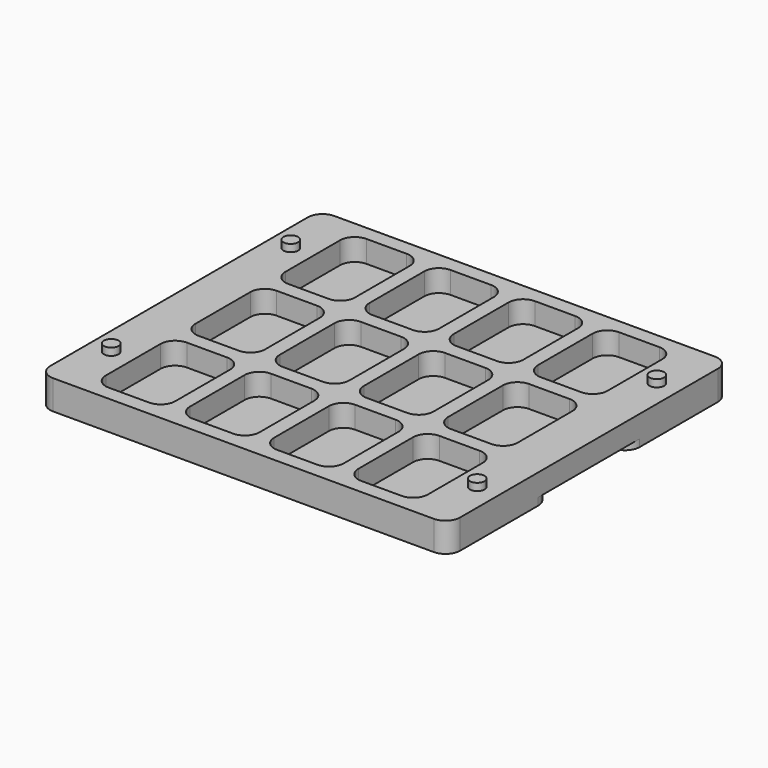
from build123d import *

# Parameters (mm, degrees)
F0_R     = 6.35
F1_DEPTH = 19.05
F2_DEPTH = 6.35
F3_DEPTH = 25.4


# Not quite as in the source:
# - a feature names something its author has since deleted; it is built from what else it names


with BuildPart() as f1:
    # F0 (on Top) → F1 (new body)
    with BuildSketch(Plane.XY):
        with BuildLine():
            Line((-165.1, -152.4), (165.1, -152.4))
            ThreePointArc((165.1, -152.4), (174.0802561211, -148.6802561211), (177.8, -139.7))
            Line((177.8, -139.7), (177.8, -55.0333333333))
            ThreePointArc((177.8, -55.0333333333), (174.0802561211, -46.0530772123), (165.1, -42.3333333333))
            ThreePointArc((165.1, -42.3333333333), (156.1197438789, -38.6135894544), (152.4, -29.6333333333))
            Line((152.4, -29.6333333333), (152.4, 29.6333333333))
            ThreePointArc((152.4, 29.6333333333), (156.1197438789, 38.6135894544), (165.1, 42.3333333333))
            ThreePointArc((165.1, 42.3333333333), (174.0802561211, 46.0530772123), (177.8, 55.0333333333))
            Line((177.8, 55.0333333333), (177.8, 139.7))
            ThreePointArc((177.8, 139.7), (174.0802561211, 148.6802561211), (165.1, 152.4))
            Line((165.1, 152.4), (-165.1, 152.4))
            ThreePointArc((-165.1, 152.4), (-174.0802561211, 148.6802561211), (-177.8, 139.7))
            Line((-177.8, 139.7), (-177.8, 55.0333333333))
            ThreePointArc((-177.8, 55.0333333333), (-174.0802561211, 46.0530772123), (-165.1, 42.3333333333))
            ThreePointArc((-165.1, 42.3333333333), (-156.1197438789, 38.6135894544), (-152.4, 29.6333333333))
            Line((-152.4, 29.6333333333), (-152.4, -42.3333333333))
            ThreePointArc((-152.4, -42.3333333333), (-156.1197438789, -51.3135894544), (-165.1, -55.0333333333))
            ThreePointArc((-165.1, -55.0333333333), (-174.0802561211, -58.7530772123), (-177.8, -67.7333333333))
            Line((-177.8, -67.7333333333), (-177.8, -139.7))
            ThreePointArc((-177.8, -139.7), (-174.0802561211, -148.6802561211), (-165.1, -152.4))
        make_face()
        with Locations((-158.75, -97.3666666667)):
            Circle(F0_R, mode=Mode.SUBTRACT)
        with BuildLine():
            ThreePointArc((-139.7, -67.7333333333), (-135.9802561211, -58.7530772123), (-127, -55.0333333333))
            Line((-127, -55.0333333333), (-92.075, -55.0333333333))
            ThreePointArc((-92.075, -55.0333333333), (-83.0947438789, -58.7530772123), (-79.375, -67.7333333333))
            Line((-79.375, -67.7333333333), (-79.375, -127))
            ThreePointArc((-79.375, -127), (-83.0947438789, -135.9802561211), (-92.075, -139.7))
            Line((-92.075, -139.7), (-127, -139.7))
            ThreePointArc((-127, -139.7), (-135.9802561211, -135.9802561211), (-139.7, -127))
            Line((-139.7, -127), (-139.7, -67.7333333333))
        make_face(mode=Mode.SUBTRACT)
        with BuildLine():
            ThreePointArc((-66.675, -67.7333333333), (-62.9552561211, -58.7530772123), (-53.975, -55.0333333333))
            Line((-53.975, -55.0333333333), (-19.05, -55.0333333333))
            ThreePointArc((-19.05, -55.0333333333), (-10.0697438789, -58.7530772123), (-6.35, -67.7333333333))
            Line((-6.35, -67.7333333333), (-6.35, -127))
            ThreePointArc((-6.35, -127), (-10.0697438789, -135.9802561211), (-19.05, -139.7))
            Line((-19.05, -139.7), (-53.975, -139.7))
            ThreePointArc((-53.975, -139.7), (-62.9552561211, -135.9802561211), (-66.675, -127))
            Line((-66.675, -127), (-66.675, -67.7333333333))
        make_face(mode=Mode.SUBTRACT)
        with BuildLine():
            Line((53.975, -139.7), (19.05, -139.7))
            ThreePointArc((19.05, -139.7), (10.0697438789, -135.9802561211), (6.35, -127))
            Line((6.35, -127), (6.35, -67.7333333333))
            ThreePointArc((6.35, -67.7333333333), (10.0697438789, -58.7530772123), (19.05, -55.0333333333))
            Line((19.05, -55.0333333333), (53.975, -55.0333333333))
            ThreePointArc((53.975, -55.0333333333), (62.9552561211, -58.7530772123), (66.675, -67.7333333333))
            Line((66.675, -67.7333333333), (66.675, -127))
            ThreePointArc((66.675, -127), (62.9552561211, -135.9802561211), (53.975, -139.7))
        make_face(mode=Mode.SUBTRACT)
        with BuildLine():
            ThreePointArc((79.375, -67.7333333333), (83.0947438789, -58.7530772123), (92.075, -55.0333333333))
            Line((92.075, -55.0333333333), (127, -55.0333333333))
            ThreePointArc((127, -55.0333333333), (135.9802561211, -58.7530772123), (139.7, -67.7333333333))
            Line((139.7, -67.7333333333), (139.7, -127))
            ThreePointArc((139.7, -127), (135.9802561211, -135.9802561211), (127, -139.7))
            Line((127, -139.7), (92.075, -139.7))
            ThreePointArc((92.075, -139.7), (83.0947438789, -135.9802561211), (79.375, -127))
            Line((79.375, -127), (79.375, -67.7333333333))
        make_face(mode=Mode.SUBTRACT)
        with Locations((158.75, -97.3666666667)):
            Circle(F0_R, mode=Mode.SUBTRACT)
        with BuildLine():
            Line((-127, 42.3333333333), (-92.075, 42.3333333333))
            ThreePointArc((-92.075, 42.3333333333), (-83.0947438789, 38.6135894544), (-79.375, 29.6333333333))
            Line((-79.375, 29.6333333333), (-79.375, -29.6333333333))
            ThreePointArc((-79.375, -29.6333333333), (-83.0947438789, -38.6135894544), (-92.075, -42.3333333333))
            Line((-92.075, -42.3333333333), (-127, -42.3333333333))
            ThreePointArc((-127, -42.3333333333), (-135.9802561211, -38.6135894544), (-139.7, -29.6333333333))
            Line((-139.7, -29.6333333333), (-139.7, 29.6333333333))
            ThreePointArc((-139.7, 29.6333333333), (-135.9802561211, 38.6135894544), (-127, 42.3333333333))
        make_face(mode=Mode.SUBTRACT)
        with BuildLine():
            Line((-53.975, 42.3333333333), (-19.05, 42.3333333333))
            ThreePointArc((-19.05, 42.3333333333), (-10.0697438789, 38.6135894544), (-6.35, 29.6333333333))
            Line((-6.35, 29.6333333333), (-6.35, -29.6333333333))
            ThreePointArc((-6.35, -29.6333333333), (-10.0697438789, -38.6135894544), (-19.05, -42.3333333333))
            Line((-19.05, -42.3333333333), (-53.975, -42.3333333333))
            ThreePointArc((-53.975, -42.3333333333), (-62.9552561211, -38.6135894544), (-66.675, -29.6333333333))
            Line((-66.675, -29.6333333333), (-66.675, 29.6333333333))
            ThreePointArc((-66.675, 29.6333333333), (-62.9552561211, 38.6135894544), (-53.975, 42.3333333333))
        make_face(mode=Mode.SUBTRACT)
        with Locations((-158.75, 97.3666666667)):
            Circle(F0_R, mode=Mode.SUBTRACT)
        with BuildLine():
            ThreePointArc((-139.7, 127), (-135.9802561211, 135.9802561211), (-127, 139.7))
            Line((-127, 139.7), (-92.075, 139.7))
            ThreePointArc((-92.075, 139.7), (-83.0947438789, 135.9802561211), (-79.375, 127))
            Line((-79.375, 127), (-79.375, 67.7333333333))
            ThreePointArc((-79.375, 67.7333333333), (-83.0947438789, 58.7530772123), (-92.075, 55.0333333333))
            Line((-92.075, 55.0333333333), (-127, 55.0333333333))
            ThreePointArc((-127, 55.0333333333), (-135.9802561211, 58.7530772123), (-139.7, 67.7333333333))
            Line((-139.7, 67.7333333333), (-139.7, 127))
        make_face(mode=Mode.SUBTRACT)
        with BuildLine():
            ThreePointArc((-66.675, 127), (-62.9552561211, 135.9802561211), (-53.975, 139.7))
            Line((-53.975, 139.7), (-19.05, 139.7))
            ThreePointArc((-19.05, 139.7), (-10.0697438789, 135.9802561211), (-6.35, 127))
            Line((-6.35, 127), (-6.35, 67.7333333333))
            ThreePointArc((-6.35, 67.7333333333), (-10.0697438789, 58.7530772123), (-19.05, 55.0333333333))
            Line((-19.05, 55.0333333333), (-53.975, 55.0333333333))
            ThreePointArc((-53.975, 55.0333333333), (-62.9552561211, 58.7530772123), (-66.675, 67.7333333333))
            Line((-66.675, 67.7333333333), (-66.675, 127))
        make_face(mode=Mode.SUBTRACT)
        with BuildLine():
            ThreePointArc((66.675, -29.6333333333), (62.9552561211, -38.6135894544), (53.975, -42.3333333333))
            Line((53.975, -42.3333333333), (19.05, -42.3333333333))
            ThreePointArc((19.05, -42.3333333333), (10.0697438789, -38.6135894544), (6.35, -29.6333333333))
            Line((6.35, -29.6333333333), (6.35, 29.6333333333))
            ThreePointArc((6.35, 29.6333333333), (10.0697438789, 38.6135894544), (19.05, 42.3333333333))
            Line((19.05, 42.3333333333), (53.975, 42.3333333333))
            ThreePointArc((53.975, 42.3333333333), (62.9552561211, 38.6135894544), (66.675, 29.6333333333))
            Line((66.675, 29.6333333333), (66.675, -29.6333333333))
        make_face(mode=Mode.SUBTRACT)
        with BuildLine():
            Line((92.075, 42.3333333333), (127, 42.3333333333))
            ThreePointArc((127, 42.3333333333), (135.9802561211, 38.6135894544), (139.7, 29.6333333333))
            Line((139.7, 29.6333333333), (139.7, -29.6333333333))
            ThreePointArc((139.7, -29.6333333333), (135.9802561211, -38.6135894544), (127, -42.3333333333))
            Line((127, -42.3333333333), (92.075, -42.3333333333))
            ThreePointArc((92.075, -42.3333333333), (83.0947438789, -38.6135894544), (79.375, -29.6333333333))
            Line((79.375, -29.6333333333), (79.375, 29.6333333333))
            ThreePointArc((79.375, 29.6333333333), (83.0947438789, 38.6135894544), (92.075, 42.3333333333))
        make_face(mode=Mode.SUBTRACT)
        with BuildLine():
            Line((53.975, 55.0333333333), (19.05, 55.0333333333))
            ThreePointArc((19.05, 55.0333333333), (10.0697438789, 58.7530772123), (6.35, 67.7333333333))
            Line((6.35, 67.7333333333), (6.35, 127))
            ThreePointArc((6.35, 127), (10.0697438789, 135.9802561211), (19.05, 139.7))
            Line((19.05, 139.7), (53.975, 139.7))
            ThreePointArc((53.975, 139.7), (62.9552561211, 135.9802561211), (66.675, 127))
            Line((66.675, 127), (66.675, 67.7333333333))
            ThreePointArc((66.675, 67.7333333333), (62.9552561211, 58.7530772123), (53.975, 55.0333333333))
        make_face(mode=Mode.SUBTRACT)
        with BuildLine():
            ThreePointArc((79.375, 127), (83.0947438789, 135.9802561211), (92.075, 139.7))
            Line((92.075, 139.7), (127, 139.7))
            ThreePointArc((127, 139.7), (135.9802561211, 135.9802561211), (139.7, 127))
            Line((139.7, 127), (139.7, 67.7333333333))
            ThreePointArc((139.7, 67.7333333333), (135.9802561211, 58.7530772123), (127, 55.0333333333))
            Line((127, 55.0333333333), (92.075, 55.0333333333))
            ThreePointArc((92.075, 55.0333333333), (83.0947438789, 58.7530772123), (79.375, 67.7333333333))
            Line((79.375, 67.7333333333), (79.375, 127))
        make_face(mode=Mode.SUBTRACT)
        with Locations((158.75, 97.3666666667)):
            Circle(F0_R, mode=Mode.SUBTRACT)
        with BuildLine():
            Line((-177.8, 55.0333333333), (-177.8, -67.7333333333))
            ThreePointArc((-177.8, -67.7333333333), (-174.0802561211, -58.7530772123), (-165.1, -55.0333333333))
            ThreePointArc((-165.1, -55.0333333333), (-156.1197438789, -51.3135894544), (-152.4, -42.3333333333))
            Line((-152.4, -42.3333333333), (-152.4, 29.6333333333))
            ThreePointArc((-152.4, 29.6333333333), (-156.1197438789, 38.6135894544), (-165.1, 42.3333333333))
            ThreePointArc((-165.1, 42.3333333333), (-174.0802561211, 46.0530772123), (-177.8, 55.0333333333))
        make_face()
        with BuildLine():
            ThreePointArc((165.1, -42.3333333333), (174.0802561211, -46.0530772123), (177.8, -55.0333333333))
            Line((177.8, -55.0333333333), (177.8, 55.0333333333))
            ThreePointArc((177.8, 55.0333333333), (174.0802561211, 46.0530772123), (165.1, 42.3333333333))
            ThreePointArc((165.1, 42.3333333333), (156.1197438789, 38.6135894544), (152.4, 29.6333333333))
            Line((152.4, 29.6333333333), (152.4, -29.6333333333))
            ThreePointArc((152.4, -29.6333333333), (156.1197438789, -38.6135894544), (165.1, -42.3333333333))
        make_face()
    extrude(amount=F1_DEPTH)

    # F0 (on Top) → F2 (join)
    with BuildSketch(Plane.XY):
        with BuildLine():
            Line((-165.1, -152.4), (165.1, -152.4))
            ThreePointArc((165.1, -152.4), (174.0802561211, -148.6802561211), (177.8, -139.7))
            Line((177.8, -139.7), (177.8, -55.0333333333))
            ThreePointArc((177.8, -55.0333333333), (174.0802561211, -46.0530772123), (165.1, -42.3333333333))
            ThreePointArc((165.1, -42.3333333333), (156.1197438789, -38.6135894544), (152.4, -29.6333333333))
            Line((152.4, -29.6333333333), (152.4, 29.6333333333))
            ThreePointArc((152.4, 29.6333333333), (156.1197438789, 38.6135894544), (165.1, 42.3333333333))
            ThreePointArc((165.1, 42.3333333333), (174.0802561211, 46.0530772123), (177.8, 55.0333333333))
            Line((177.8, 55.0333333333), (177.8, 139.7))
            ThreePointArc((177.8, 139.7), (174.0802561211, 148.6802561211), (165.1, 152.4))
            Line((165.1, 152.4), (-165.1, 152.4))
            ThreePointArc((-165.1, 152.4), (-174.0802561211, 148.6802561211), (-177.8, 139.7))
            Line((-177.8, 139.7), (-177.8, 55.0333333333))
            ThreePointArc((-177.8, 55.0333333333), (-174.0802561211, 46.0530772123), (-165.1, 42.3333333333))
            ThreePointArc((-165.1, 42.3333333333), (-156.1197438789, 38.6135894544), (-152.4, 29.6333333333))
            Line((-152.4, 29.6333333333), (-152.4, -42.3333333333))
            ThreePointArc((-152.4, -42.3333333333), (-156.1197438789, -51.3135894544), (-165.1, -55.0333333333))
            ThreePointArc((-165.1, -55.0333333333), (-174.0802561211, -58.7530772123), (-177.8, -67.7333333333))
            Line((-177.8, -67.7333333333), (-177.8, -139.7))
            ThreePointArc((-177.8, -139.7), (-174.0802561211, -148.6802561211), (-165.1, -152.4))
        make_face()
        with Locations((-158.75, -97.3666666667)):
            Circle(F0_R, mode=Mode.SUBTRACT)
        with BuildLine():
            ThreePointArc((-139.7, -67.7333333333), (-135.9802561211, -58.7530772123), (-127, -55.0333333333))
            Line((-127, -55.0333333333), (-92.075, -55.0333333333))
            ThreePointArc((-92.075, -55.0333333333), (-83.0947438789, -58.7530772123), (-79.375, -67.7333333333))
            Line((-79.375, -67.7333333333), (-79.375, -127))
            ThreePointArc((-79.375, -127), (-83.0947438789, -135.9802561211), (-92.075, -139.7))
            Line((-92.075, -139.7), (-127, -139.7))
            ThreePointArc((-127, -139.7), (-135.9802561211, -135.9802561211), (-139.7, -127))
            Line((-139.7, -127), (-139.7, -67.7333333333))
        make_face(mode=Mode.SUBTRACT)
        with BuildLine():
            ThreePointArc((-66.675, -67.7333333333), (-62.9552561211, -58.7530772123), (-53.975, -55.0333333333))
            Line((-53.975, -55.0333333333), (-19.05, -55.0333333333))
            ThreePointArc((-19.05, -55.0333333333), (-10.0697438789, -58.7530772123), (-6.35, -67.7333333333))
            Line((-6.35, -67.7333333333), (-6.35, -127))
            ThreePointArc((-6.35, -127), (-10.0697438789, -135.9802561211), (-19.05, -139.7))
            Line((-19.05, -139.7), (-53.975, -139.7))
            ThreePointArc((-53.975, -139.7), (-62.9552561211, -135.9802561211), (-66.675, -127))
            Line((-66.675, -127), (-66.675, -67.7333333333))
        make_face(mode=Mode.SUBTRACT)
        with BuildLine():
            Line((53.975, -139.7), (19.05, -139.7))
            ThreePointArc((19.05, -139.7), (10.0697438789, -135.9802561211), (6.35, -127))
            Line((6.35, -127), (6.35, -67.7333333333))
            ThreePointArc((6.35, -67.7333333333), (10.0697438789, -58.7530772123), (19.05, -55.0333333333))
            Line((19.05, -55.0333333333), (53.975, -55.0333333333))
            ThreePointArc((53.975, -55.0333333333), (62.9552561211, -58.7530772123), (66.675, -67.7333333333))
            Line((66.675, -67.7333333333), (66.675, -127))
            ThreePointArc((66.675, -127), (62.9552561211, -135.9802561211), (53.975, -139.7))
        make_face(mode=Mode.SUBTRACT)
        with BuildLine():
            ThreePointArc((79.375, -67.7333333333), (83.0947438789, -58.7530772123), (92.075, -55.0333333333))
            Line((92.075, -55.0333333333), (127, -55.0333333333))
            ThreePointArc((127, -55.0333333333), (135.9802561211, -58.7530772123), (139.7, -67.7333333333))
            Line((139.7, -67.7333333333), (139.7, -127))
            ThreePointArc((139.7, -127), (135.9802561211, -135.9802561211), (127, -139.7))
            Line((127, -139.7), (92.075, -139.7))
            ThreePointArc((92.075, -139.7), (83.0947438789, -135.9802561211), (79.375, -127))
            Line((79.375, -127), (79.375, -67.7333333333))
        make_face(mode=Mode.SUBTRACT)
        with Locations((158.75, -97.3666666667)):
            Circle(F0_R, mode=Mode.SUBTRACT)
        with BuildLine():
            Line((-127, 42.3333333333), (-92.075, 42.3333333333))
            ThreePointArc((-92.075, 42.3333333333), (-83.0947438789, 38.6135894544), (-79.375, 29.6333333333))
            Line((-79.375, 29.6333333333), (-79.375, -29.6333333333))
            ThreePointArc((-79.375, -29.6333333333), (-83.0947438789, -38.6135894544), (-92.075, -42.3333333333))
            Line((-92.075, -42.3333333333), (-127, -42.3333333333))
            ThreePointArc((-127, -42.3333333333), (-135.9802561211, -38.6135894544), (-139.7, -29.6333333333))
            Line((-139.7, -29.6333333333), (-139.7, 29.6333333333))
            ThreePointArc((-139.7, 29.6333333333), (-135.9802561211, 38.6135894544), (-127, 42.3333333333))
        make_face(mode=Mode.SUBTRACT)
        with BuildLine():
            Line((-53.975, 42.3333333333), (-19.05, 42.3333333333))
            ThreePointArc((-19.05, 42.3333333333), (-10.0697438789, 38.6135894544), (-6.35, 29.6333333333))
            Line((-6.35, 29.6333333333), (-6.35, -29.6333333333))
            ThreePointArc((-6.35, -29.6333333333), (-10.0697438789, -38.6135894544), (-19.05, -42.3333333333))
            Line((-19.05, -42.3333333333), (-53.975, -42.3333333333))
            ThreePointArc((-53.975, -42.3333333333), (-62.9552561211, -38.6135894544), (-66.675, -29.6333333333))
            Line((-66.675, -29.6333333333), (-66.675, 29.6333333333))
            ThreePointArc((-66.675, 29.6333333333), (-62.9552561211, 38.6135894544), (-53.975, 42.3333333333))
        make_face(mode=Mode.SUBTRACT)
        with Locations((-158.75, 97.3666666667)):
            Circle(F0_R, mode=Mode.SUBTRACT)
        with BuildLine():
            ThreePointArc((-139.7, 127), (-135.9802561211, 135.9802561211), (-127, 139.7))
            Line((-127, 139.7), (-92.075, 139.7))
            ThreePointArc((-92.075, 139.7), (-83.0947438789, 135.9802561211), (-79.375, 127))
            Line((-79.375, 127), (-79.375, 67.7333333333))
            ThreePointArc((-79.375, 67.7333333333), (-83.0947438789, 58.7530772123), (-92.075, 55.0333333333))
            Line((-92.075, 55.0333333333), (-127, 55.0333333333))
            ThreePointArc((-127, 55.0333333333), (-135.9802561211, 58.7530772123), (-139.7, 67.7333333333))
            Line((-139.7, 67.7333333333), (-139.7, 127))
        make_face(mode=Mode.SUBTRACT)
        with BuildLine():
            ThreePointArc((-66.675, 127), (-62.9552561211, 135.9802561211), (-53.975, 139.7))
            Line((-53.975, 139.7), (-19.05, 139.7))
            ThreePointArc((-19.05, 139.7), (-10.0697438789, 135.9802561211), (-6.35, 127))
            Line((-6.35, 127), (-6.35, 67.7333333333))
            ThreePointArc((-6.35, 67.7333333333), (-10.0697438789, 58.7530772123), (-19.05, 55.0333333333))
            Line((-19.05, 55.0333333333), (-53.975, 55.0333333333))
            ThreePointArc((-53.975, 55.0333333333), (-62.9552561211, 58.7530772123), (-66.675, 67.7333333333))
            Line((-66.675, 67.7333333333), (-66.675, 127))
        make_face(mode=Mode.SUBTRACT)
        with BuildLine():
            ThreePointArc((66.675, -29.6333333333), (62.9552561211, -38.6135894544), (53.975, -42.3333333333))
            Line((53.975, -42.3333333333), (19.05, -42.3333333333))
            ThreePointArc((19.05, -42.3333333333), (10.0697438789, -38.6135894544), (6.35, -29.6333333333))
            Line((6.35, -29.6333333333), (6.35, 29.6333333333))
            ThreePointArc((6.35, 29.6333333333), (10.0697438789, 38.6135894544), (19.05, 42.3333333333))
            Line((19.05, 42.3333333333), (53.975, 42.3333333333))
            ThreePointArc((53.975, 42.3333333333), (62.9552561211, 38.6135894544), (66.675, 29.6333333333))
            Line((66.675, 29.6333333333), (66.675, -29.6333333333))
        make_face(mode=Mode.SUBTRACT)
        with BuildLine():
            Line((92.075, 42.3333333333), (127, 42.3333333333))
            ThreePointArc((127, 42.3333333333), (135.9802561211, 38.6135894544), (139.7, 29.6333333333))
            Line((139.7, 29.6333333333), (139.7, -29.6333333333))
            ThreePointArc((139.7, -29.6333333333), (135.9802561211, -38.6135894544), (127, -42.3333333333))
            Line((127, -42.3333333333), (92.075, -42.3333333333))
            ThreePointArc((92.075, -42.3333333333), (83.0947438789, -38.6135894544), (79.375, -29.6333333333))
            Line((79.375, -29.6333333333), (79.375, 29.6333333333))
            ThreePointArc((79.375, 29.6333333333), (83.0947438789, 38.6135894544), (92.075, 42.3333333333))
        make_face(mode=Mode.SUBTRACT)
        with BuildLine():
            Line((53.975, 55.0333333333), (19.05, 55.0333333333))
            ThreePointArc((19.05, 55.0333333333), (10.0697438789, 58.7530772123), (6.35, 67.7333333333))
            Line((6.35, 67.7333333333), (6.35, 127))
            ThreePointArc((6.35, 127), (10.0697438789, 135.9802561211), (19.05, 139.7))
            Line((19.05, 139.7), (53.975, 139.7))
            ThreePointArc((53.975, 139.7), (62.9552561211, 135.9802561211), (66.675, 127))
            Line((66.675, 127), (66.675, 67.7333333333))
            ThreePointArc((66.675, 67.7333333333), (62.9552561211, 58.7530772123), (53.975, 55.0333333333))
        make_face(mode=Mode.SUBTRACT)
        with BuildLine():
            ThreePointArc((79.375, 127), (83.0947438789, 135.9802561211), (92.075, 139.7))
            Line((92.075, 139.7), (127, 139.7))
            ThreePointArc((127, 139.7), (135.9802561211, 135.9802561211), (139.7, 127))
            Line((139.7, 127), (139.7, 67.7333333333))
            ThreePointArc((139.7, 67.7333333333), (135.9802561211, 58.7530772123), (127, 55.0333333333))
            Line((127, 55.0333333333), (92.075, 55.0333333333))
            ThreePointArc((92.075, 55.0333333333), (83.0947438789, 58.7530772123), (79.375, 67.7333333333))
            Line((79.375, 67.7333333333), (79.375, 127))
        make_face(mode=Mode.SUBTRACT)
        with Locations((158.75, 97.3666666667)):
            Circle(F0_R, mode=Mode.SUBTRACT)
        with BuildLine():
            Line((-92.075, 139.7), (-127, 139.7))
            ThreePointArc((-127, 139.7), (-135.9802561211, 135.9802561211), (-139.7, 127))
            Line((-139.7, 127), (-139.7, 67.7333333333))
            ThreePointArc((-139.7, 67.7333333333), (-135.9802561211, 58.7530772123), (-127, 55.0333333333))
            Line((-127, 55.0333333333), (-92.075, 55.0333333333))
            ThreePointArc((-92.075, 55.0333333333), (-83.0947438789, 58.7530772123), (-79.375, 67.7333333333))
            Line((-79.375, 67.7333333333), (-79.375, 127))
            ThreePointArc((-79.375, 127), (-83.0947438789, 135.9802561211), (-92.075, 139.7))
        make_face()
        with BuildLine():
            ThreePointArc((-79.375, 29.6333333333), (-83.0947438789, 38.6135894544), (-92.075, 42.3333333333))
            Line((-92.075, 42.3333333333), (-127, 42.3333333333))
            ThreePointArc((-127, 42.3333333333), (-135.9802561211, 38.6135894544), (-139.7, 29.6333333333))
            Line((-139.7, 29.6333333333), (-139.7, -29.6333333333))
            ThreePointArc((-139.7, -29.6333333333), (-135.9802561211, -38.6135894544), (-127, -42.3333333333))
            Line((-127, -42.3333333333), (-92.075, -42.3333333333))
            ThreePointArc((-92.075, -42.3333333333), (-83.0947438789, -38.6135894544), (-79.375, -29.6333333333))
            Line((-79.375, -29.6333333333), (-79.375, 29.6333333333))
        make_face()
        with BuildLine():
            Line((-92.075, -55.0333333333), (-127, -55.0333333333))
            ThreePointArc((-127, -55.0333333333), (-135.9802561211, -58.7530772123), (-139.7, -67.7333333333))
            Line((-139.7, -67.7333333333), (-139.7, -127))
            ThreePointArc((-139.7, -127), (-135.9802561211, -135.9802561211), (-127, -139.7))
            Line((-127, -139.7), (-92.075, -139.7))
            ThreePointArc((-92.075, -139.7), (-83.0947438789, -135.9802561211), (-79.375, -127))
            Line((-79.375, -127), (-79.375, -67.7333333333))
            ThreePointArc((-79.375, -67.7333333333), (-83.0947438789, -58.7530772123), (-92.075, -55.0333333333))
        make_face()
        with BuildLine():
            Line((-19.05, -55.0333333333), (-53.975, -55.0333333333))
            ThreePointArc((-53.975, -55.0333333333), (-62.9552561211, -58.7530772123), (-66.675, -67.7333333333))
            Line((-66.675, -67.7333333333), (-66.675, -127))
            ThreePointArc((-66.675, -127), (-62.9552561211, -135.9802561211), (-53.975, -139.7))
            Line((-53.975, -139.7), (-19.05, -139.7))
            ThreePointArc((-19.05, -139.7), (-10.0697438789, -135.9802561211), (-6.35, -127))
            Line((-6.35, -127), (-6.35, -67.7333333333))
            ThreePointArc((-6.35, -67.7333333333), (-10.0697438789, -58.7530772123), (-19.05, -55.0333333333))
        make_face()
        with BuildLine():
            Line((-19.05, 139.7), (-53.975, 139.7))
            ThreePointArc((-53.975, 139.7), (-62.9552561211, 135.9802561211), (-66.675, 127))
            Line((-66.675, 127), (-66.675, 67.7333333333))
            ThreePointArc((-66.675, 67.7333333333), (-62.9552561211, 58.7530772123), (-53.975, 55.0333333333))
            Line((-53.975, 55.0333333333), (-19.05, 55.0333333333))
            ThreePointArc((-19.05, 55.0333333333), (-10.0697438789, 58.7530772123), (-6.35, 67.7333333333))
            Line((-6.35, 67.7333333333), (-6.35, 127))
            ThreePointArc((-6.35, 127), (-10.0697438789, 135.9802561211), (-19.05, 139.7))
        make_face()
        with BuildLine():
            ThreePointArc((6.35, 67.7333333333), (10.0697438789, 58.7530772123), (19.05, 55.0333333333))
            Line((19.05, 55.0333333333), (53.975, 55.0333333333))
            ThreePointArc((53.975, 55.0333333333), (62.9552561211, 58.7530772123), (66.675, 67.7333333333))
            Line((66.675, 67.7333333333), (66.675, 127))
            ThreePointArc((66.675, 127), (62.9552561211, 135.9802561211), (53.975, 139.7))
            Line((53.975, 139.7), (19.05, 139.7))
            ThreePointArc((19.05, 139.7), (10.0697438789, 135.9802561211), (6.35, 127))
            Line((6.35, 127), (6.35, 67.7333333333))
        make_face()
        with BuildLine():
            Line((19.05, -42.3333333333), (53.975, -42.3333333333))
            ThreePointArc((53.975, -42.3333333333), (62.9552561211, -38.6135894544), (66.675, -29.6333333333))
            Line((66.675, -29.6333333333), (66.675, 29.6333333333))
            ThreePointArc((66.675, 29.6333333333), (62.9552561211, 38.6135894544), (53.975, 42.3333333333))
            Line((53.975, 42.3333333333), (19.05, 42.3333333333))
            ThreePointArc((19.05, 42.3333333333), (10.0697438789, 38.6135894544), (6.35, 29.6333333333))
            Line((6.35, 29.6333333333), (6.35, -29.6333333333))
            ThreePointArc((6.35, -29.6333333333), (10.0697438789, -38.6135894544), (19.05, -42.3333333333))
        make_face()
        with BuildLine():
            ThreePointArc((6.35, -127), (10.0697438789, -135.9802561211), (19.05, -139.7))
            Line((19.05, -139.7), (53.975, -139.7))
            ThreePointArc((53.975, -139.7), (62.9552561211, -135.9802561211), (66.675, -127))
            Line((66.675, -127), (66.675, -67.7333333333))
            ThreePointArc((66.675, -67.7333333333), (62.9552561211, -58.7530772123), (53.975, -55.0333333333))
            Line((53.975, -55.0333333333), (19.05, -55.0333333333))
            ThreePointArc((19.05, -55.0333333333), (10.0697438789, -58.7530772123), (6.35, -67.7333333333))
            Line((6.35, -67.7333333333), (6.35, -127))
        make_face()
        with BuildLine():
            Line((127, -55.0333333333), (92.075, -55.0333333333))
            ThreePointArc((92.075, -55.0333333333), (83.0947438789, -58.7530772123), (79.375, -67.7333333333))
            Line((79.375, -67.7333333333), (79.375, -127))
            ThreePointArc((79.375, -127), (83.0947438789, -135.9802561211), (92.075, -139.7))
            Line((92.075, -139.7), (127, -139.7))
            ThreePointArc((127, -139.7), (135.9802561211, -135.9802561211), (139.7, -127))
            Line((139.7, -127), (139.7, -67.7333333333))
            ThreePointArc((139.7, -67.7333333333), (135.9802561211, -58.7530772123), (127, -55.0333333333))
        make_face()
        with BuildLine():
            ThreePointArc((139.7, 29.6333333333), (135.9802561211, 38.6135894544), (127, 42.3333333333))
            Line((127, 42.3333333333), (92.075, 42.3333333333))
            ThreePointArc((92.075, 42.3333333333), (83.0947438789, 38.6135894544), (79.375, 29.6333333333))
            Line((79.375, 29.6333333333), (79.375, -29.6333333333))
            ThreePointArc((79.375, -29.6333333333), (83.0947438789, -38.6135894544), (92.075, -42.3333333333))
            Line((92.075, -42.3333333333), (127, -42.3333333333))
            ThreePointArc((127, -42.3333333333), (135.9802561211, -38.6135894544), (139.7, -29.6333333333))
            Line((139.7, -29.6333333333), (139.7, 29.6333333333))
        make_face()
        with BuildLine():
            Line((127, 139.7), (92.075, 139.7))
            ThreePointArc((92.075, 139.7), (83.0947438789, 135.9802561211), (79.375, 127))
            Line((79.375, 127), (79.375, 67.7333333333))
            ThreePointArc((79.375, 67.7333333333), (83.0947438789, 58.7530772123), (92.075, 55.0333333333))
            Line((92.075, 55.0333333333), (127, 55.0333333333))
            ThreePointArc((127, 55.0333333333), (135.9802561211, 58.7530772123), (139.7, 67.7333333333))
            Line((139.7, 67.7333333333), (139.7, 127))
            ThreePointArc((139.7, 127), (135.9802561211, 135.9802561211), (127, 139.7))
        make_face()
        with BuildLine():
            ThreePointArc((-6.35, 29.6333333333), (-10.0697438789, 38.6135894544), (-19.05, 42.3333333333))
            Line((-19.05, 42.3333333333), (-53.975, 42.3333333333))
            ThreePointArc((-53.975, 42.3333333333), (-62.9552561211, 38.6135894544), (-66.675, 29.6333333333))
            Line((-66.675, 29.6333333333), (-66.675, -29.6333333333))
            ThreePointArc((-66.675, -29.6333333333), (-62.9552561211, -38.6135894544), (-53.975, -42.3333333333))
            Line((-53.975, -42.3333333333), (-19.05, -42.3333333333))
            ThreePointArc((-19.05, -42.3333333333), (-10.0697438789, -38.6135894544), (-6.35, -29.6333333333))
            Line((-6.35, -29.6333333333), (-6.35, 29.6333333333))
        make_face()
    extrude(amount=-F2_DEPTH)

    # F0 (on Top) → F3 (join)
    with BuildSketch(Plane.XY):
        with Locations((158.75, -97.3666666667)):
            Circle(F0_R)
        with Locations((158.75, 97.3666666667)):
            Circle(F0_R)
        with Locations((-158.75, -97.3666666667)):
            Circle(F0_R)
        with Locations((-158.75, 97.3666666667)):
            Circle(F0_R)
    extrude(amount=F3_DEPTH)


solid = f1.part
